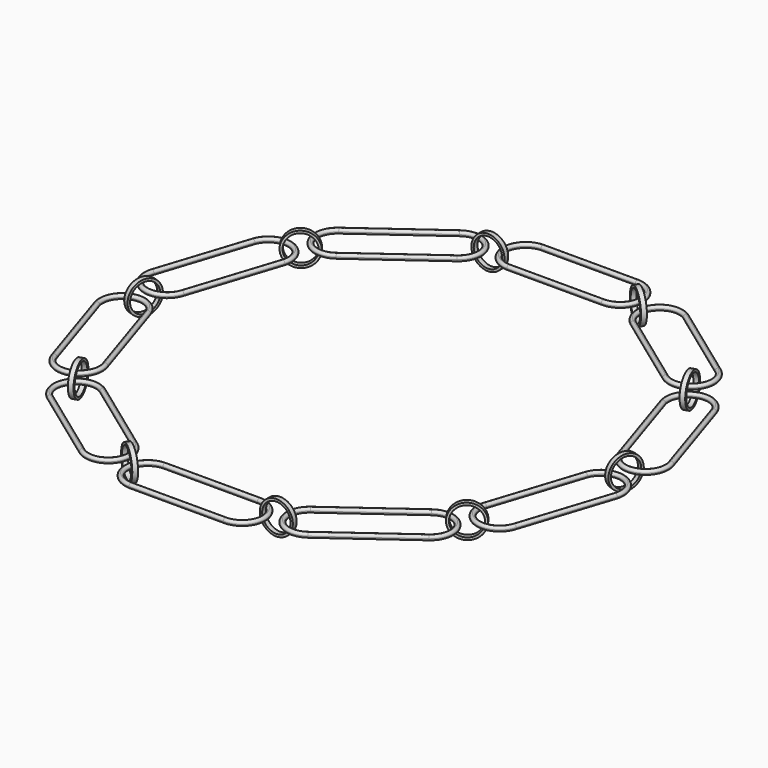
from build123d import *

# Parameters (mm, degrees)
F1_DEPTH = 1
F2_R     = 0.49999
F4_R     = 3.5
F4_R_2   = 3
F5_DEPTH = 0.5
F7_COUNT = 10


# Not quite as in the source:
# - a fillet or chamfer is up to 0.001 mm smaller than in the source, because OpenCascade refuses the exact size


with BuildPart() as f1:
    # F0 (on Top) → F1 (new body)
    with BuildSketch(Plane.XY):
        with BuildLine():
            Line((10, -45), (-10, -45))
            ThreePointArc((-10, -45), (-15, -50), (-10, -55))
            Line((-10, -55), (10, -55))
            ThreePointArc((10, -55), (15, -50), (10, -45))
        make_face()
        with BuildLine():
            ThreePointArc((-10, -53.9999999106), (-13.9999999106, -50), (-10, -46.0000000894))
            Line((-10, -46.0000000894), (10, -46.0000000894))
            ThreePointArc((10, -46.0000000894), (13.9999999106, -50), (10, -53.9999999106))
            Line((10, -53.9999999106), (-10, -53.9999999106))
        make_face(mode=Mode.SUBTRACT)
    extrude(amount=F1_DEPTH)

    # F2 (radius 0.5 in the source; OpenCascade refuses exactly that, so slightly less here)
    f2_edges = [f1.edges().sort_by_distance(p)[0] for p in [
        (0, -46, 1),
        (0, -46, 0),
        (15, -50, 1),
        (15, -50, 0),
    ]]
    fillet(f2_edges, radius=F2_R)


with BuildPart() as f5:
    # F4 (on offset) → F5 (new body, symmetric)
    with BuildSketch(Plane.XZ.offset(48)):
        with Locations((16, 0.5)):
            Circle(F4_R)
        with Locations((16, 0.5)):
            Circle(F4_R_2, mode=Mode.SUBTRACT)
    extrude(amount=F5_DEPTH, both=True)


with BuildPart() as f7_1:
    # F7: instance of F1
    add(f1.part.rotate(Axis((0, 0, -0.0070165843), (0, 0, -1)), 1 * 360 / F7_COUNT))


with BuildPart() as f7_2:
    # F7: instance of F1
    add(f1.part.rotate(Axis((0, 0, -0.0070165843), (0, 0, -1)), 2 * 360 / F7_COUNT))


with BuildPart() as f7_3:
    # F7: instance of F1
    add(f1.part.rotate(Axis((0, 0, -0.0070165843), (0, 0, -1)), 3 * 360 / F7_COUNT))


with BuildPart() as f7_4:
    # F7: instance of F1
    add(f1.part.rotate(Axis((0, 0, -0.0070165843), (0, 0, -1)), 4 * 360 / F7_COUNT))


with BuildPart() as f7_5:
    # F7: instance of F1
    add(f1.part.rotate(Axis((0, 0, -0.0070165843), (0, 0, -1)), 5 * 360 / F7_COUNT))


with BuildPart() as f7_6:
    # F7: instance of F1
    add(f1.part.rotate(Axis((0, 0, -0.0070165843), (0, 0, -1)), 6 * 360 / F7_COUNT))


with BuildPart() as f7_7:
    # F7: instance of F1
    add(f1.part.rotate(Axis((0, 0, -0.0070165843), (0, 0, -1)), 7 * 360 / F7_COUNT))


with BuildPart() as f7_8:
    # F7: instance of F1
    add(f1.part.rotate(Axis((0, 0, -0.0070165843), (0, 0, -1)), 8 * 360 / F7_COUNT))


with BuildPart() as f7_9:
    # F7: instance of F1
    add(f1.part.rotate(Axis((0, 0, -0.0070165843), (0, 0, -1)), 9 * 360 / F7_COUNT))


with BuildPart() as f7_10:
    # F7: instance of F5
    add(f5.part.rotate(Axis((0, 0, -0.0070165843), (0, 0, -1)), 1 * 360 / F7_COUNT))


with BuildPart() as f7_11:
    # F7: instance of F5
    add(f5.part.rotate(Axis((0, 0, -0.0070165843), (0, 0, -1)), 2 * 360 / F7_COUNT))


with BuildPart() as f7_12:
    # F7: instance of F5
    add(f5.part.rotate(Axis((0, 0, -0.0070165843), (0, 0, -1)), 3 * 360 / F7_COUNT))


with BuildPart() as f7_13:
    # F7: instance of F5
    add(f5.part.rotate(Axis((0, 0, -0.0070165843), (0, 0, -1)), 4 * 360 / F7_COUNT))


with BuildPart() as f7_14:
    # F7: instance of F5
    add(f5.part.rotate(Axis((0, 0, -0.0070165843), (0, 0, -1)), 5 * 360 / F7_COUNT))


with BuildPart() as f7_15:
    # F7: instance of F5
    add(f5.part.rotate(Axis((0, 0, -0.0070165843), (0, 0, -1)), 6 * 360 / F7_COUNT))


with BuildPart() as f7_16:
    # F7: instance of F5
    add(f5.part.rotate(Axis((0, 0, -0.0070165843), (0, 0, -1)), 7 * 360 / F7_COUNT))


with BuildPart() as f7_17:
    # F7: instance of F5
    add(f5.part.rotate(Axis((0, 0, -0.0070165843), (0, 0, -1)), 8 * 360 / F7_COUNT))


with BuildPart() as f7_18:
    # F7: instance of F5
    add(f5.part.rotate(Axis((0, 0, -0.0070165843), (0, 0, -1)), 9 * 360 / F7_COUNT))


solid = Compound([f1.part, f5.part, f7_1.part, f7_2.part, f7_3.part, f7_4.part, f7_5.part, f7_6.part, f7_7.part, f7_8.part, f7_9.part, f7_10.part, f7_11.part, f7_12.part, f7_13.part, f7_14.part, f7_15.part, f7_16.part, f7_17.part, f7_18.part])
